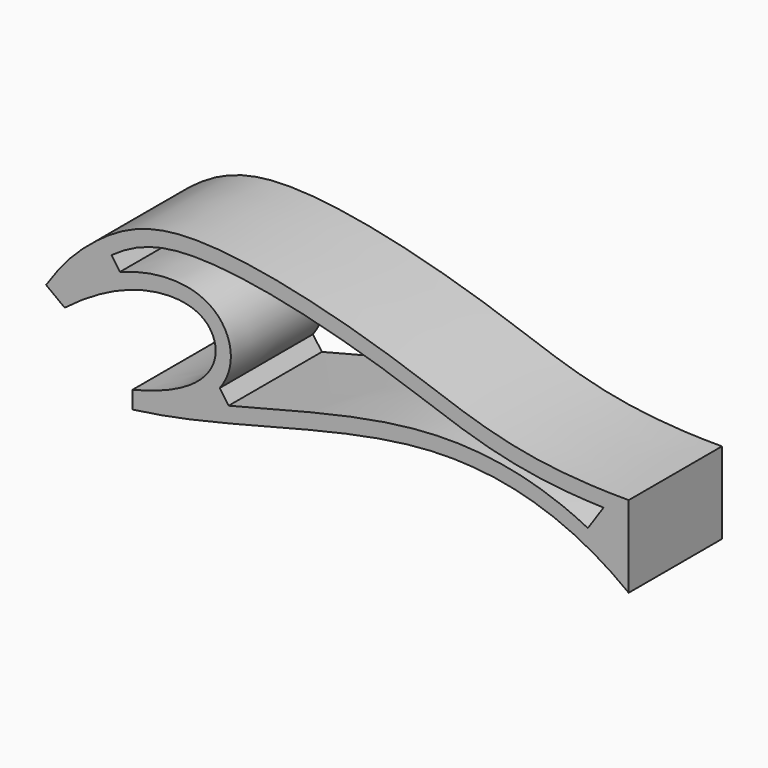
from build123d import *

# Parameters (mm, degrees)
F1_DEPTH = 10


# Not quite as in the source:
# - ends of sketch curves that miss each other by under 0.0002 mm in the source are joined
# - the dataset's text gives a spline's control points without its knots; the knots are read off the source's solid


with BuildPart() as f1:
    # F0 (on Front) → F1 (new body)
    with BuildSketch(Plane.XZ):
        with BuildLine():
            add(Edge.make_bspline(
                [(-25, 0), (-23.5353633761, 2.2088184487), (-21.0062414356, 4.7820689833), (-13.8192409759, 9.2564060733), (7.7997359992, 3.8412558696), (15.1413595304, 0), (25, 0)],
                knots=[0, 0, 0, 0, 0.176877597, 0.369937696, 0.6842072965, 1, 1, 1, 1], degree=3))
            Line((-25, 0), (-23.4013824598, -1.2018410711))
            add(Edge.make_bspline(
                [(-23.4013824598, -1.2018410711), (-20.7961176234, 0.8105589099), (-16.2151711553, 3.1186773641), (-9.4114614583, 2.2080487325), (-10.1234289262, -3.6913444212), (-17.5727587193, -5.5)],
                knots=[0, 0, 0, 0, 0.3577339943, 0.6237725059, 1, 1, 1, 1], degree=3))
            Line((-17.5727587193, -5.5), (-17.5727587193, -7))
            add(Edge.make_bspline(
                [(-17.5727587193, -7), (-9.5416165347, -6.0225988186), (7.3368503694, 0.6895433506), (19.9003461748, -3.1075021252), (25, -7)],
                knots=[0, 0, 0, 0, 0.5421146173, 1, 1, 1, 1], degree=3))
            Line((25, -7), (25, 0))
        make_face()
        with BuildLine():
            Line((-18.6626309713, 3.0437360985), (-19.37718185, 4.085818865))
            add(Edge.make_bspline(
                [(-19.37718185, 4.085818865), (-19.2351469903, 4.1884605588), (-18.8222001915, 4.476962296), (-18.1021841377, 4.9225532755), (-17.1701670507, 5.3871128646), (-16.1314871306, 5.7748903375), (-14.9555077334, 6.0692782464), (-13.6178958905, 6.247793332), (-12.0666825691, 6.2914734797), (-9.766124237, 6.1813777311), (-6.5603478578, 5.7549083191), (-2.4752672416, 4.8953532484), (0.9014991571, 3.9920741444), (3.4564214075, 3.2193291581), (5.26222423, 2.6315789588), (6.9431379993, 2.0470359162), (9.1025443307, 1.2805575784), (11.7720133473, 0.3721732526), (15.3081169524, -0.5345270337), (18.9866204844, -1.0692247139), (21.7134251241, -1.2326363335), (22.8392417874, -1.2675846816)],
                knots=[0.2019930137, 0.2019930137, 0.2019930137, 0.2019930137, 0.21875, 0.25, 0.28125, 0.3125, 0.34375, 0.375, 0.40625, 0.4375, 0.5, 0.5625, 0.625, 0.65625, 0.6875, 0.71875, 0.75, 0.8125, 0.875, 0.9375, 0.9762819293, 0.9762819293, 0.9762819293, 0.9762819293], degree=3))
            Line((22.8392417874, -1.2675846816), (21.4982855177, -3.2547442942))
            add(Edge.make_bspline(
                [(-9.3299190223, -4.026907105), (-8.3286212906, -3.7769416853), (-5.3537756133, -3.0091078031), (-1.3560313783, -1.9756906659), (2.573556358, -1.1515681653), (5.4810935362, -0.6888547782), (8.3362134892, -0.4422460036), (11.1009276127, -0.4565682672), (13.7766541289, -0.7274180604), (17.2253435912, -1.4336165841), (19.7627439648, -2.3827163169), (21.4155417012, -3.2126347425), (21.4982855177, -3.2547442942)],
                knots=[0.1858417609, 0.1858417609, 0.1858417609, 0.1858417609, 0.25, 0.375, 0.4375, 0.5, 0.5625, 0.625, 0.6875, 0.75, 0.875, 0.8816021473, 0.8816021473, 0.8816021473, 0.8816021473], degree=3))
            Line((-9.3299190223, -4.026907105), (-10.1023896224, -2.948806003))
            add(Edge.make_bspline(
                [(-18.6626309713, 3.0437360985), (-18.5725818066, 3.0780117008), (-17.99215712, 3.2926858769), (-16.9176681891, 3.6175018842), (-15.4366583445, 3.8846431492), (-13.9518702414, 3.9539138632), (-12.5024766902, 3.7725777912), (-11.354806853, 3.3399679954), (-10.5294772781, 2.7650699008), (-9.8062415879, 2.0269023954), (-9.2987612179, 1.0630274045), (-9.1161197289, -0.0633099369), (-9.1716226788, -0.9572739007), (-9.435887283, -1.860198698), (-9.7938332887, -2.5206201828), (-10.0472997743, -2.8755973617), (-10.1023896224, -2.948806003)],
                knots=[0.2385136662, 0.2385136662, 0.2385136662, 0.2385136662, 0.25, 0.3125, 0.375, 0.4375, 0.5, 0.5625, 0.59375, 0.625, 0.6875, 0.71875, 0.75, 0.78125, 0.8125, 0.8207073926, 0.8207073926, 0.8207073926, 0.8207073926], degree=3))
        make_face(mode=Mode.SUBTRACT)
    extrude(amount=F1_DEPTH)


solid = f1.part
